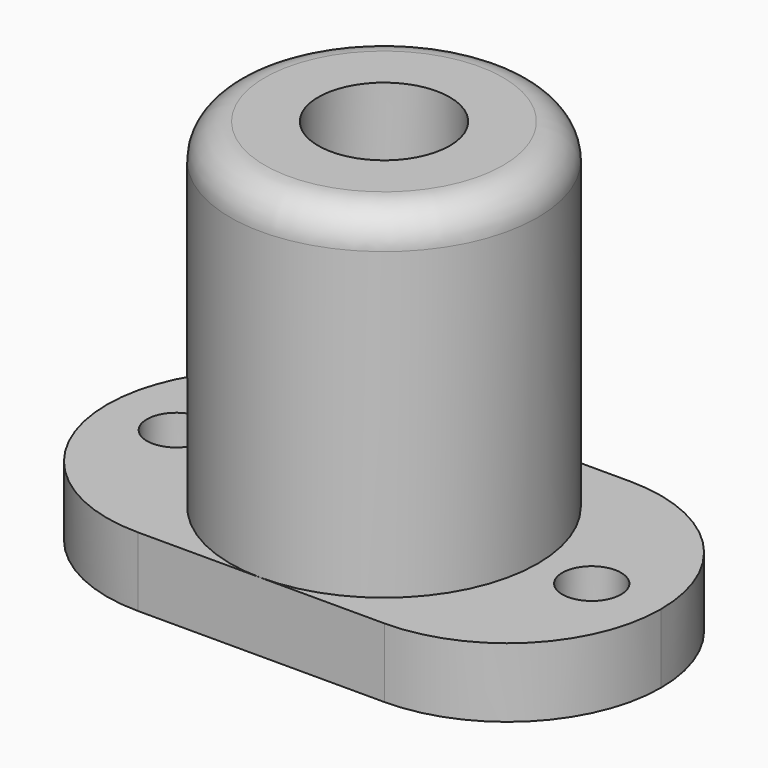
from build123d import *

# Parameters (mm, degrees)
F0_W     = 40
F0_H     = 22.2
F0_R     = 2.125
F0_R_2   = 7.825
F1_DEPTH = 5
F2_R     = 11.1
F2_R_2   = 7.825
F3_DEPTH = 19.5
F4_R     = 11.1
F4_R_2   = 4.75
F5_DEPTH = 5
F6_R     = 11.09999
F7_R     = 2.5


# Not quite as in the source:
# - a fillet or chamfer is up to 0.001 mm smaller than in the source, because OpenCascade refuses the exact size


with BuildPart() as f1:
    # F0 (on Top) → F1 (new body)
    with BuildSketch(Plane.XY):
        Rectangle(F0_W, F0_H)
        with Locations((-15, 0)):
            Circle(F0_R, mode=Mode.SUBTRACT)
        Circle(F0_R_2, mode=Mode.SUBTRACT)
        with Locations((15, 0)):
            Circle(F0_R, mode=Mode.SUBTRACT)
    extrude(amount=F1_DEPTH)

    # F2 (on face) → F3 (join)
    with BuildSketch(Plane.XY.offset(5)):
        Circle(F2_R)
        Circle(F2_R_2, mode=Mode.SUBTRACT)
    extrude(amount=F3_DEPTH)

    # F4 (on face) → F5 (join)
    with BuildSketch(Plane.XY.offset(24.5)):
        Circle(F4_R)
        Circle(F4_R_2, mode=Mode.SUBTRACT)
    extrude(amount=F5_DEPTH)

    # F6 (radius 11.1 in the source; OpenCascade refuses exactly that, so slightly less here)
    f6_edges = [f1.edges().sort_by_distance(p)[0] for p in [
        (-20, 11.1, 2.5),
        (-20, -11.1, 2.5),
        (20, -11.1, 2.5),
        (20, 11.1, 2.5),
    ]]
    fillet(f6_edges, radius=F6_R)

    # F7
    f7_edges = [f1.edges().sort_by_distance(p)[0] for p in [
        (-11.1, 0, 29.5),
    ]]
    fillet(f7_edges, radius=F7_R)


solid = f1.part
